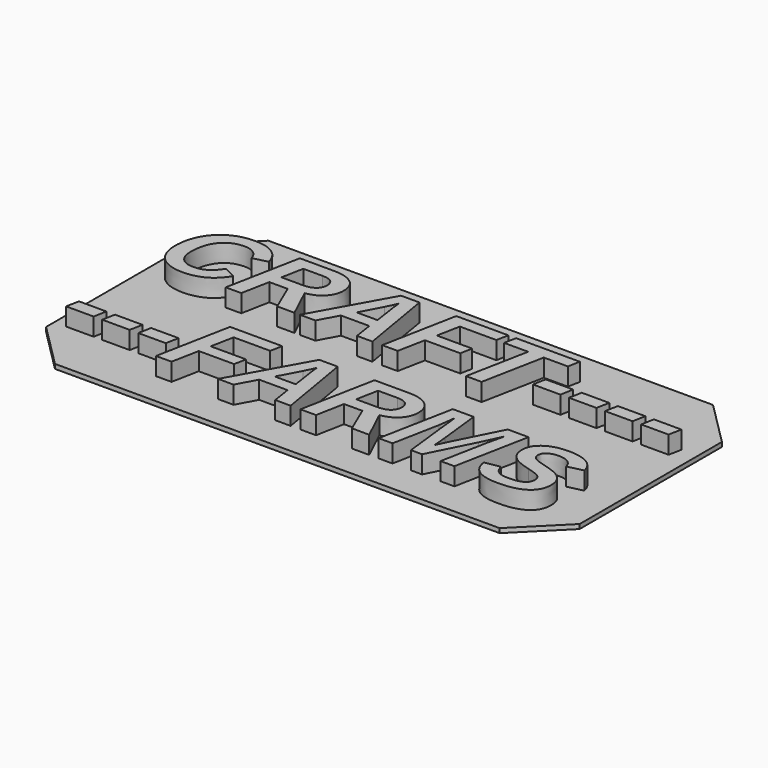
from build123d import *

# Parameters (mm, degrees)
F0_TEXT_SIZE = 30.9455166076
F1_DEPTH     = 6.35
F2_DEPTH     = 1.27


# Not quite as in the source:
# - Text() gives the source's letters only with a copy of the font that has no kerning and outlines rounded to 1/6400 em; it was checked with that copy


with BuildPart() as f1:
    # F0 (on Top) → F1 (new body)
    with BuildSketch(Plane.XY):
        with Locations((-73.66, 6.9292280425)):
            Text('CRAFT----', F0_TEXT_SIZE, font='Arimo', font_style=FontStyle.BOLDITALIC, text_align=(TextAlign.LEFT, TextAlign.BOTTOM))
        with Locations((-73.66, -28.6581160562)):
            Text('---FARMS', F0_TEXT_SIZE, font='Arimo', font_style=FontStyle.BOLDITALIC, text_align=(TextAlign.LEFT, TextAlign.BOTTOM))
    extrude(amount=F1_DEPTH)

    # F0 (on Top) → F2 (join)
    with BuildSketch(Plane.XY):
        Polygon((63.5, 38.1), (-63.5, 38.1), (-76.2, 25.4), (-76.2, -25.4), (-63.5, -38.1), (63.5, -38.1), (76.2, -25.4), (76.2, 25.4), align=None)
        Polygon((-64.9565734541, -22.4786832086), (-72.8138335303, -22.4786832086), (-72.1030536957, -18.7893974006), (-64.2457936195, -18.7893974006), align=None, mode=Mode.SUBTRACT)
        Polygon((-54.6526834712, -22.4786832086), (-62.5099435473, -22.4786832086), (-61.7991637127, -18.7893974006), (-53.9419036366, -18.7893974006), align=None, mode=Mode.SUBTRACT)
        Polygon((-44.3487934882, -22.4786832086), (-52.2060535644, -22.4786832086), (-51.4952737298, -18.7893974006), (-43.6380136537, -18.7893974006), align=None, mode=Mode.SUBTRACT)
        Polygon((-23.8473887357, -10.8112564002), (-34.2866653538, -10.8112564002), (-35.5728383878, -17.4016843902), (-25.4768635946, -17.4016843902), (-26.1441262964, -20.8443731128), (-36.2352658527, -20.8443731128), (-37.7632007352, -28.6581160562), (-42.2019482736, -28.6581160562), (-38.0774911382, -7.3685676776), (-23.1801260339, -7.3685676776), align=None, mode=Mode.SUBTRACT)
        Polygon((-3.7376381778, -28.6581160562), (-8.1473742943, -28.6581160562), (-8.9790350532, -23.218474465), (-17.0925626887, -23.218474465), (-20.0372220034, -28.6581160562), (-24.4808047788, -28.6581160562), (-12.5909570697, -7.3685676776), (-7.3302192464, -7.3685676776), align=None, mode=Mode.SUBTRACT)
        with BuildLine():
            Line((18.6881908888, -28.6581160562), (13.7610844164, -28.6581160562))
            Line((13.7610844164, -28.6581160562), (10.289384272, -20.5881055534))
            Line((10.289384272, -20.5881055534), (5.0576578706, -20.5881055534))
            Line((5.0576578706, -20.5881055534), (3.5007115662, -28.6581160562))
            Line((3.5007115662, -28.6581160562), (-0.9525416831, -28.6581160562))
            Line((-0.9525416831, -28.6581160562), (3.1864211632, -7.3685676776))
            Line((3.1864211632, -7.3685676776), (13.02129316, -7.3685676776))
            add(Edge.make_bspline(
                [(13.02129316, -7.3685676776), (15.4244059341, -7.3685676776), (17.1384974399, -8.108358934)],
                knots=[0, 0, 0, 1, 1, 1], degree=2))
            add(Edge.make_bspline(
                [(17.1384974399, -8.108358934), (18.8525889458, -8.8481501904), (19.7446901667, -10.2237751083)],
                knots=[0, 0, 0, 1, 1, 1], degree=2))
            add(Edge.make_bspline(
                [(19.7446901667, -10.2237751083), (20.6367913877, -11.5994000263), (20.6367913877, -13.4561310227)],
                knots=[0, 0, 0, 1, 1, 1], degree=2))
            add(Edge.make_bspline(
                [(20.6367913877, -13.4561310227), (20.6367913877, -15.9511132992), (18.9976460549, -17.6893809899)],
                knots=[0, 0, 0, 1, 1, 1], degree=2))
            add(Edge.make_bspline(
                [(18.9976460549, -17.6893809899), (17.3585007221, -19.4276486806), (14.5492280425, -19.848314297)],
                knots=[0, 0, 0, 1, 1, 1], degree=2))
            Line((14.5492280425, -19.848314297), (18.6881908888, -28.6581160562))
        make_face(mode=Mode.SUBTRACT)
        with BuildLine():
            Line((43.0336090324, -28.6581160562), (39.0735499541, -28.6581160562))
            Line((39.0735499541, -28.6581160562), (41.6700722069, -15.2983563083))
            add(Edge.make_bspline(
                [(41.6700722069, -15.2983563083), (42.0665616384, -13.3352500985), (42.7918471839, -10.4341079165)],
                knots=[0, 0, 0, 1, 1, 1], degree=2))
            Line((42.7918471839, -10.4341079165), (41.7474359984, -12.7163397663))
            add(Edge.make_bspline(
                [(41.7474359984, -12.7163397663), (40.5531324669, -15.346708678), (40.0260916371, -16.3282617829)],
                knots=[0, 0, 0, 1, 1, 1], degree=2))
            Line((40.0260916371, -16.3282617829), (33.7983064199, -28.6581160562))
            Line((33.7983064199, -28.6581160562), (30.6263909676, -28.6581160562))
            Line((30.6263909676, -28.6581160562), (29.2048312984, -16.2847446501))
            add(Edge.make_bspline(
                [(29.2048312984, -16.2847446501), (28.7358133123, -11.8846790075), (28.6004266772, -10.4341079165)],
                knots=[0, 0, 0, 1, 1, 1], degree=2))
            add(Edge.make_bspline(
                [(28.6004266772, -10.4341079165), (28.1797610608, -14.1233937246), (27.9525049232, -15.2548391755)],
                knots=[0, 0, 0, 1, 1, 1], degree=2))
            Line((27.9525049232, -15.2548391755), (25.3511474334, -28.6581160562))
            Line((25.3511474334, -28.6581160562), (21.395923592, -28.6581160562))
            Line((21.395923592, -28.6581160562), (25.5348864382, -7.3685676776))
            Line((25.5348864382, -7.3685676776), (31.5015688591, -7.3685676776))
            Line((31.5015688591, -7.3685676776), (32.8312590259, -19.2729210975))
            Line((32.8312590259, -19.2729210975), (33.2084075095, -23.4457306026))
            add(Edge.make_bspline(
                [(33.2084075095, -23.4457306026), (33.7547892871, -22.2369213601), (34.2238072732, -21.2553682552)],
                knots=[0, 0, 0, 1, 1, 1], degree=2))
            add(Edge.make_bspline(
                [(34.2238072732, -21.2553682552), (34.6928252593, -20.2738151503), (41.2349008796, -7.3685676776)],
                knots=[0, 0, 0, 1, 1, 1], degree=2))
            Line((41.2349008796, -7.3685676776), (47.1725718787, -7.3685676776))
            Line((47.1725718787, -7.3685676776), (43.0336090324, -28.6581160562))
        make_face(mode=Mode.SUBTRACT)
        with BuildLine():
            add(Edge.make_bspline(
                [(63.0659957989, -27.246226861), (60.5565078115, -28.9627359853), (55.6922594197, -28.9627359853)],
                knots=[0, 0, 0, 1, 1, 1], degree=2))
            add(Edge.make_bspline(
                [(55.6922594197, -28.9627359853), (51.6596717868, -28.9627359853), (49.5442556124, -27.5339234607)],
                knots=[0, 0, 0, 1, 1, 1], degree=2))
            add(Edge.make_bspline(
                [(49.5442556124, -27.5339234607), (47.4288394381, -26.1051109361), (47.0033385847, -23.1411106735)],
                knots=[0, 0, 0, 1, 1, 1], degree=2))
            Line((47.0033385847, -23.1411106735), (51.3695575686, -22.4013194171))
            add(Edge.make_bspline(
                [(51.3695575686, -22.4013194171), (51.6886832086, -24.0791466457), (52.7838643823, -24.8503669424)],
                knots=[0, 0, 0, 1, 1, 1], degree=2))
            add(Edge.make_bspline(
                [(52.7838643823, -24.8503669424), (53.879045556, -25.6215872391), (55.9968793488, -25.6215872391)],
                knots=[0, 0, 0, 1, 1, 1], degree=2))
            add(Edge.make_bspline(
                [(55.9968793488, -25.6215872391), (61.2092648024, -25.6215872391), (61.2092648024, -22.6140698438)],
                knots=[0, 0, 0, 1, 1, 1], degree=2))
            add(Edge.make_bspline(
                [(61.2092648024, -22.6140698438), (61.2092648024, -21.4052606013), (60.3026578706, -20.7017336222)],
                knots=[0, 0, 0, 1, 1, 1], degree=2))
            add(Edge.make_bspline(
                [(60.3026578706, -20.7017336222), (59.3960509387, -19.998206643), (56.7028239464, -19.3212734672)],
                knots=[0, 0, 0, 1, 1, 1], degree=2))
            add(Edge.make_bspline(
                [(56.7028239464, -19.3212734672), (53.9225626887, -18.5814822108), (52.5856196665, -17.7788328738)],
                knots=[0, 0, 0, 1, 1, 1], degree=2))
            add(Edge.make_bspline(
                [(52.5856196665, -17.7788328738), (51.2486766443, -16.9761835368), (50.5475672837, -15.820561901)],
                knots=[0, 0, 0, 1, 1, 1], degree=2))
            add(Edge.make_bspline(
                [(50.5475672837, -15.820561901), (49.8464579231, -14.6649402652), (49.8464579231, -12.9871130366)],
                knots=[0, 0, 0, 1, 1, 1], degree=2))
            add(Edge.make_bspline(
                [(49.8464579231, -12.9871130366), (49.8464579231, -10.3132269923), (52.2181416568, -8.6813345149)],
                knots=[0, 0, 0, 1, 1, 1], degree=2))
            add(Edge.make_bspline(
                [(52.2181416568, -8.6813345149), (54.5898253906, -7.0494420375), (58.5015320993, -7.0494420375)],
                knots=[0, 0, 0, 1, 1, 1], degree=2))
            add(Edge.make_bspline(
                [(58.5015320993, -7.0494420375), (62.0989484049, -7.0494420375), (64.2748050414, -8.3573736379)],
                knots=[0, 0, 0, 1, 1, 1], degree=2))
            add(Edge.make_bspline(
                [(64.2748050414, -8.3573736379), (66.4506616778, -9.6653052383), (66.9486910857, -12.1747932257)],
                knots=[0, 0, 0, 1, 1, 1], degree=2))
            Line((66.9486910857, -12.1747932257), (62.5969778128, -13.1853577524))
            add(Edge.make_bspline(
                [(62.5969778128, -13.1853577524), (62.2633464619, -11.8266561638), (61.1536595773, -11.0167539714)],
                knots=[0, 0, 0, 1, 1, 1], degree=2))
            add(Edge.make_bspline(
                [(61.1536595773, -11.0167539714), (60.0439726927, -10.2068517789), (58.2597702508, -10.2068517789)],
                knots=[0, 0, 0, 1, 1, 1], degree=2))
            add(Edge.make_bspline(
                [(58.2597702508, -10.2068517789), (56.3885335434, -10.2068517789), (55.3151109361, -10.910378758)],
                knots=[0, 0, 0, 1, 1, 1], degree=2))
            add(Edge.make_bspline(
                [(55.3151109361, -10.910378758), (54.2416883287, -11.6139057372), (54.2416883287, -12.8372206906)],
                knots=[0, 0, 0, 1, 1, 1], degree=2))
            add(Edge.make_bspline(
                [(54.2416883287, -12.8372206906), (54.2416883287, -13.5480005251), (54.6357601418, -14.046029933)],
                knots=[0, 0, 0, 1, 1, 1], degree=2))
            add(Edge.make_bspline(
                [(54.6357601418, -14.046029933), (55.0298319548, -14.5440593409), (55.7841289221, -14.9139549691)],
                knots=[0, 0, 0, 1, 1, 1], degree=2))
            add(Edge.make_bspline(
                [(55.7841289221, -14.9139549691), (56.5384258895, -15.2838505973), (58.7771406065, -15.8882552186)],
                knots=[0, 0, 0, 1, 1, 1], degree=2))
            add(Edge.make_bspline(
                [(58.7771406065, -15.8882552186), (61.1754181436, -16.5555179204), (62.323786924, -17.1357463568)],
                knots=[0, 0, 0, 1, 1, 1], degree=2))
            add(Edge.make_bspline(
                [(62.323786924, -17.1357463568), (63.4721557043, -17.7159747932), (64.1611769726, -18.4412603387)],
                knots=[0, 0, 0, 1, 1, 1], degree=2))
            add(Edge.make_bspline(
                [(64.1611769726, -18.4412603387), (64.8501982408, -19.1665458842), (65.2128410135, -20.1045818564)],
                knots=[0, 0, 0, 1, 1, 1], degree=2))
            add(Edge.make_bspline(
                [(65.2128410135, -20.1045818564), (65.5754837863, -21.0426178285), (65.5754837863, -22.2659327819)],
                knots=[0, 0, 0, 1, 1, 1], degree=2))
            add(Edge.make_bspline(
                [(65.5754837863, -22.2659327819), (65.5754837863, -25.5297177366), (63.0659957989, -27.246226861)],
                knots=[0, 0, 0, 1, 1, 1], degree=2))
        make_face(mode=Mode.SUBTRACT)
        with BuildLine():
            add(Edge.make_bspline(
                [(-65.5222961796, 22.4938558488), (-67.6014480767, 19.9553564395), (-67.6014480767, 15.5891374557)],
                knots=[0, 0, 0, 1, 1, 1], degree=2))
            add(Edge.make_bspline(
                [(-67.6014480767, 15.5891374557), (-67.6014480767, 12.973274255), (-66.3080221872, 11.5444617303)],
                knots=[0, 0, 0, 1, 1, 1], degree=2))
            add(Edge.make_bspline(
                [(-66.3080221872, 11.5444617303), (-65.0145962978, 10.1156492057), (-62.6163187607, 10.1156492057)],
                knots=[0, 0, 0, 1, 1, 1], degree=2))
            add(Edge.make_bspline(
                [(-62.6163187607, 10.1156492057), (-58.5934016017, 10.1156492057), (-56.296664041, 14.0176854405)],
                knots=[0, 0, 0, 1, 1, 1], degree=2))
            Line((-56.296664041, 14.0176854405), (-52.8684810293, 12.2479887095))
            add(Edge.make_bspline(
                [(-52.8684810293, 12.2479887095), (-56.0403964816, 6.6246081134), (-62.9161034528, 6.6246081134)],
                knots=[0, 0, 0, 1, 1, 1], degree=2))
            add(Edge.make_bspline(
                [(-62.9161034528, 6.6246081134), (-65.8027399239, 6.6246081134), (-67.8963975318, 7.7149540502)],
                knots=[0, 0, 0, 1, 1, 1], degree=2))
            add(Edge.make_bspline(
                [(-67.8963975318, 7.7149540502), (-69.9900551398, 8.8052999869), (-71.0683129841, 10.8215938033)],
                knots=[0, 0, 0, 1, 1, 1], degree=2))
            add(Edge.make_bspline(
                [(-71.0683129841, 10.8215938033), (-72.1465708284, 12.8378876198), (-72.1465708284, 15.5262793751)],
                knots=[0, 0, 0, 1, 1, 1], degree=2))
            add(Edge.make_bspline(
                [(-72.1465708284, 15.5262793751), (-72.1465708284, 19.3364461074), (-70.5606131023, 22.3342930288)],
                knots=[0, 0, 0, 1, 1, 1], degree=2))
            add(Edge.make_bspline(
                [(-70.5606131023, 22.3342930288), (-68.9746553761, 25.3321399501), (-66.1267008008, 26.9350210056)],
                knots=[0, 0, 0, 1, 1, 1], degree=2))
            add(Edge.make_bspline(
                [(-66.1267008008, 26.9350210056), (-63.2787462255, 28.5379020612), (-59.6523184981, 28.5379020612)],
                knots=[0, 0, 0, 1, 1, 1], degree=2))
            add(Edge.make_bspline(
                [(-59.6523184981, 28.5379020612), (-56.1757831167, 28.5379020612), (-53.9467388736, 27.0486490744)],
                knots=[0, 0, 0, 1, 1, 1], degree=2))
            add(Edge.make_bspline(
                [(-53.9467388736, 27.0486490744), (-51.7176946304, 25.5593960877), (-50.9488919522, 22.614736773)],
                knots=[0, 0, 0, 1, 1, 1], degree=2))
            Line((-50.9488919522, 22.614736773), (-55.0878547985, 21.5413141657))
            add(Edge.make_bspline(
                [(-55.0878547985, 21.5413141657), (-55.5278613627, 23.1562833136), (-56.765682027, 24.0943192858)],
                knots=[0, 0, 0, 1, 1, 1], degree=2))
            add(Edge.make_bspline(
                [(-56.765682027, 24.0943192858), (-58.0035026913, 25.032355258), (-59.7877051333, 25.032355258)],
                knots=[0, 0, 0, 1, 1, 1], degree=2))
            add(Edge.make_bspline(
                [(-59.7877051333, 25.032355258), (-63.4431442825, 25.032355258), (-65.5222961796, 22.4938558488)],
                knots=[0, 0, 0, 1, 1, 1], degree=2))
        make_face(mode=Mode.SUBTRACT)
        with BuildLine():
            Line((-31.1244203755, 6.9292280425), (-36.0515268478, 6.9292280425))
            Line((-36.0515268478, 6.9292280425), (-39.5232269923, 14.9992385454))
            Line((-39.5232269923, 14.9992385454), (-44.7549533937, 14.9992385454))
            Line((-44.7549533937, 14.9992385454), (-46.311899698, 6.9292280425))
            Line((-46.311899698, 6.9292280425), (-50.7651529474, 6.9292280425))
            Line((-50.7651529474, 6.9292280425), (-46.6261901011, 28.2187764212))
            Line((-46.6261901011, 28.2187764212), (-36.7913181042, 28.2187764212))
            add(Edge.make_bspline(
                [(-36.7913181042, 28.2187764212), (-34.3882053302, 28.2187764212), (-32.6741138243, 27.4789851648)],
                knots=[0, 0, 0, 1, 1, 1], degree=2))
            add(Edge.make_bspline(
                [(-32.6741138243, 27.4789851648), (-30.9600223185, 26.7391939084), (-30.0679210975, 25.3635689904)],
                knots=[0, 0, 0, 1, 1, 1], degree=2))
            add(Edge.make_bspline(
                [(-30.0679210975, 25.3635689904), (-29.1758198766, 23.9879440725), (-29.1758198766, 22.131213076)],
                knots=[0, 0, 0, 1, 1, 1], degree=2))
            add(Edge.make_bspline(
                [(-29.1758198766, 22.131213076), (-29.1758198766, 19.6362307995), (-30.8149652094, 17.8979631088)],
                knots=[0, 0, 0, 1, 1, 1], degree=2))
            add(Edge.make_bspline(
                [(-30.8149652094, 17.8979631088), (-32.4541105422, 16.1596954181), (-35.2633832217, 15.7390298018)],
                knots=[0, 0, 0, 1, 1, 1], degree=2))
            Line((-35.2633832217, 15.7390298018), (-31.1244203755, 6.9292280425))
        make_face(mode=Mode.SUBTRACT)
        Polygon((-8.853318892, 6.9292280425), (-13.2630550085, 6.9292280425), (-14.0947157674, 12.3688696337), (-22.2082434029, 12.3688696337), (-25.1529027176, 6.9292280425), (-29.596485493, 6.9292280425), (-17.7066377839, 28.2187764212), (-12.4458999606, 28.2187764212), align=None, mode=Mode.SUBTRACT)
        Polygon((12.2863371406, 24.7760876986), (1.8470605225, 24.7760876986), (0.5608874885, 18.1856597085), (10.6568622817, 18.1856597085), (9.9895995799, 14.742970986), (-0.1015399764, 14.742970986), (-1.6294748589, 6.9292280425), (-6.0682223973, 6.9292280425), (-1.9437652619, 28.2187764212), (12.9535998425, 28.2187764212), align=None, mode=Mode.SUBTRACT)
        Polygon((32.7007076277, 24.7760876986), (25.8104949455, 24.7760876986), (22.3339595641, 6.9292280425), (17.8758710779, 6.9292280425), (21.3524064592, 24.7760876986), (14.476699488, 24.7760876986), (15.1439621898, 28.2187764212), (33.3631350926, 28.2187764212), align=None, mode=Mode.SUBTRACT)
        Polygon((39.890705002, 13.1086608901), (32.0334449258, 13.1086608901), (32.7442247604, 16.7979466982), (40.6014848365, 16.7979466982), align=None, mode=Mode.SUBTRACT)
        Polygon((50.1945949849, 13.1086608901), (42.3373349088, 13.1086608901), (43.0481147433, 16.7979466982), (50.9053748195, 16.7979466982), align=None, mode=Mode.SUBTRACT)
        Polygon((60.4984849678, 13.1086608901), (52.6412248917, 13.1086608901), (53.3520047263, 16.7979466982), (61.2092648024, 16.7979466982), align=None, mode=Mode.SUBTRACT)
        Polygon((70.8023749508, 13.1086608901), (62.9451148746, 13.1086608901), (63.6558947092, 16.7979466982), (71.5131547853, 16.7979466982), align=None, mode=Mode.SUBTRACT)
        with BuildLine():
            Line((-44.073184981, 18.4757739267), (-38.1355139819, 18.4757739267))
            add(Edge.make_bspline(
                [(-38.1355139819, 18.4757739267), (-35.9451516345, 18.4757739267), (-34.8185414205, 19.3582046738)],
                knots=[0, 0, 0, 1, 1, 1], degree=2))
            add(Edge.make_bspline(
                [(-34.8185414205, 19.3582046738), (-33.6919312065, 20.2406354208), (-33.6919312065, 21.8749455166)],
                knots=[0, 0, 0, 1, 1, 1], degree=2))
            add(Edge.make_bspline(
                [(-33.6919312065, 21.8749455166), (-33.6919312065, 23.2771642379), (-34.651725745, 24.0193731128)],
                knots=[0, 0, 0, 1, 1, 1], degree=2))
            add(Edge.make_bspline(
                [(-34.651725745, 24.0193731128), (-35.6115202836, 24.7615819877), (-37.3473703558, 24.7615819877)],
                knots=[0, 0, 0, 1, 1, 1], degree=2))
            Line((-37.3473703558, 24.7615819877), (-42.8498700276, 24.7615819877))
            Line((-42.8498700276, 24.7615819877), (-44.073184981, 18.4757739267))
        make_face()
        with BuildLine():
            add(Edge.make_bspline(
                [(-15.4534173559, 22.5518786924), (-15.7241906262, 24.5923486937), (-15.7241906262, 24.9404857555)],
                knots=[0, 0, 0, 1, 1, 1], degree=2))
            add(Edge.make_bspline(
                [(-15.7241906262, 24.9404857555), (-16.0433162662, 23.9734383616), (-17.208608376, 21.7395588814)],
                knots=[0, 0, 0, 1, 1, 1], degree=2))
            Line((-17.208608376, 21.7395588814), (-20.4095352501, 15.7245240908))
            Line((-20.4095352501, 15.7245240908), (-14.4428528292, 15.7245240908))
            Line((-14.4428528292, 15.7245240908), (-15.4534173559, 22.5518786924))
        make_face()
        with BuildLine():
            add(Edge.make_bspline(
                [(-10.3377366417, -13.0354654063), (-10.608509912, -10.994995405), (-10.608509912, -10.6468583432)],
                knots=[0, 0, 0, 1, 1, 1], degree=2))
            add(Edge.make_bspline(
                [(-10.608509912, -10.6468583432), (-10.9276355521, -11.6139057372), (-12.0929276618, -13.8477852173)],
                knots=[0, 0, 0, 1, 1, 1], degree=2))
            Line((-12.0929276618, -13.8477852173), (-15.2938545359, -19.8628200079))
            Line((-15.2938545359, -19.8628200079), (-9.327172115, -19.8628200079))
            Line((-9.327172115, -19.8628200079), (-10.3377366417, -13.0354654063))
        make_face()
        with BuildLine():
            Line((5.7394262833, -17.111570172), (11.6770972824, -17.111570172))
            add(Edge.make_bspline(
                [(11.6770972824, -17.111570172), (13.8674596298, -17.111570172), (14.9940698438, -16.229139425)],
                knots=[0, 0, 0, 1, 1, 1], degree=2))
            add(Edge.make_bspline(
                [(14.9940698438, -16.229139425), (16.1206800578, -15.346708678), (16.1206800578, -13.7123985821)],
                knots=[0, 0, 0, 1, 1, 1], degree=2))
            add(Edge.make_bspline(
                [(16.1206800578, -13.7123985821), (16.1206800578, -12.3101798608), (15.1608855192, -11.567970986)],
                knots=[0, 0, 0, 1, 1, 1], degree=2))
            add(Edge.make_bspline(
                [(15.1608855192, -11.567970986), (14.2010909807, -10.8257621111), (12.4652409085, -10.8257621111)],
                knots=[0, 0, 0, 1, 1, 1], degree=2))
            Line((12.4652409085, -10.8257621111), (6.9627412367, -10.8257621111))
            Line((6.9627412367, -10.8257621111), (5.7394262833, -17.111570172))
        make_face()
    extrude(amount=F2_DEPTH)


solid = f1.part
